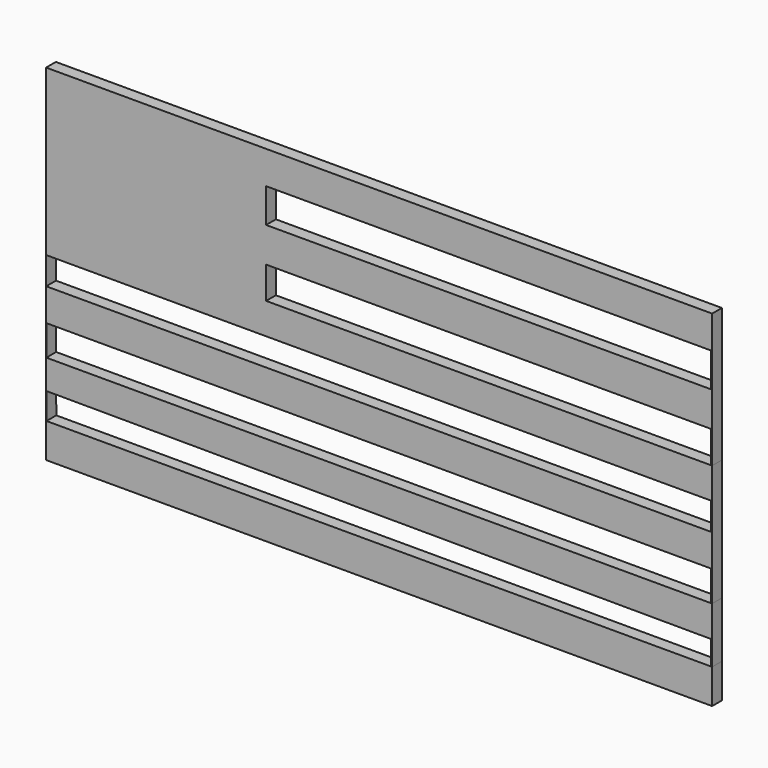
from build123d import *

# Parameters (mm, degrees)
F0_W     = 0.1980072791
F0_H     = 7.1694856525
F0_W_2   = 92.4687646329
F0_H_2   = 6.8283765789
F0_H_3   = 6.473645713
F0_H_4   = 5.7075782395
F0_H_5   = 7.0958843866
F0_H_6   = 7.2461878881
F0_H_7   = 6.6423406824
F1_DEPTH = 1.27


# Not quite as in the source:
# - a feature names something its author has since deleted; it is built from what else it names


with BuildPart() as f1:
    # F0 (on Front) → F1 (new body, symmetric)
    with BuildSketch(Plane.XZ):
        Polygon((-69.1910094554, 0), (-69.1910094554, -37.5021121278), (-69.0906792879, -37.5021121278), (-69.1058018093, -30.3326264753), (-69.1173589099, -24.8534827961), (-69.130230695, -18.7510560639), (-69.1435495608, -12.4366714017), (-69.1577431668, -5.7075782395), (-69.1697821021, 0), align=None)
        Polygon((-69.1058018093, -30.3326264753), (-69.0906792879, -37.5021121278), (68.9930021763, -37.5021121278), (68.9930021763, -30.3326264753), align=None)
        Polygon((-69.1910094554, 34.2864352491), (-69.1910094554, 0), (-69.1697821021, 0), (-23.4757624567, 0), (-23.4757624567, 6.473645713), (-23.4757624567, 13.1159863955), (-23.4757624567, 20.3621742836), (-23.4757624567, 27.4580586702), (-23.4757624567, 34.2864352491), align=None)
        with Locations((69.0920058158, -33.9173693016)):
            Rectangle(F0_W, F0_H)
        Polygon((68.9930021763, -25.3095924286), (68.9930021763, -30.3326264753), (69.1910094554, -30.3326264753), (69.1910094554, -25.3102463479), align=None)
        Polygon((-69.130230695, -18.7510560639), (-69.1173589099, -24.8534827961), (68.9930021763, -25.3095924286), (68.9930021763, -18.7510560639), align=None)
        with Locations((22.7586198598, 30.8722469596)):
            Rectangle(F0_W_2, F0_H_2)
        with Locations((22.7586198598, 3.2368228565)):
            Rectangle(F0_W_2, F0_H_3)
        Polygon((68.9930021763, -5.7075782395), (-69.1577431668, -5.7075782395), (-69.1435495608, -12.4366714017), (68.9930021763, -12.4186396162), align=None)
        Polygon((68.9930021763, -18.7510560639), (68.9930021763, -25.3095924286), (69.1910094554, -25.3102463479), (69.1910094554, -18.7510560639), align=None)
        with Locations((69.0920058158, 30.8722469596)):
            Rectangle(F0_W, F0_H_2)
        with Locations((69.0920058158, 3.2368228565)):
            Rectangle(F0_W, F0_H_3)
        with Locations((69.0920058158, -2.8537891197)):
            Rectangle(F0_W, F0_H_4)
        Polygon((69.1910094554, -5.7075782395), (68.9930021763, -5.7075782395), (68.9930021763, -12.4186396162), (69.1910094554, -12.4186137691), align=None)
        Polygon((68.9930021763, -12.4186396162), (68.9930021763, -18.7510560639), (69.1910094554, -18.7510560639), (69.1910094554, -12.4186137691), align=None)
        with Locations((69.0920058158, 23.9101164769)):
            Rectangle(F0_W, F0_H_5)
        with Locations((22.7586198598, 16.7390803395)):
            Rectangle(F0_W_2, F0_H_6)
        with Locations((69.0920058158, 9.7948160542)):
            Rectangle(F0_W, F0_H_7)
        with Locations((69.0920058158, 16.7390803395)):
            Rectangle(F0_W, F0_H_6)
    extrude(amount=F1_DEPTH, both=True)


solid = f1.part
